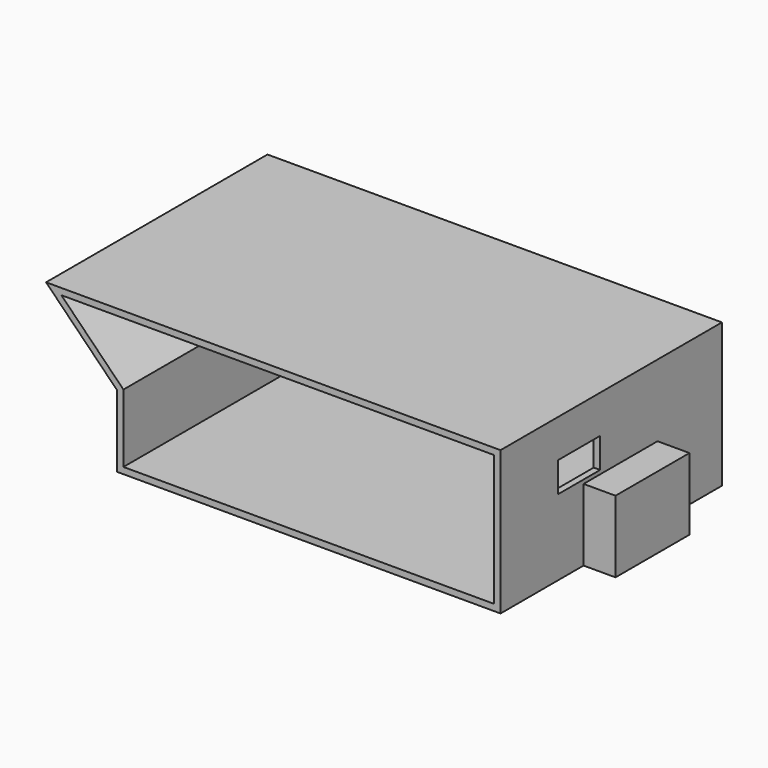
from build123d import *

# Parameters (mm, degrees)
F0_W     = 24
F0_H     = 28.575
F1_DEPTH = 54.991
F2_T     = -2.54
F3_W     = 18.5978077352
F3_H     = 17.8960040212
F4_DEPTH = 76.2
F5_W     = 36.7379160598
F5_H     = 28.575
F6_DEPTH = 12.7
F7_W     = 20.9140316583
F7_H     = 11.9311325252
F8_DEPTH = 25.4


# Not quite as in the source:
# - a feature of the source that left no trace in its solid (it failed there, or was rolled back) is left out


with BuildPart() as f1:
    # F0 (on Front) → F1 (new body, symmetric)
    with BuildSketch(Plane.XZ):
        Polygon((-76.2, -28.575), (76.2, -28.575), (76.2, 28.575), (0, 28.575), (28.2, 0), (-52.2, 0), (-76.2, 0), align=None)
        Polygon((-104.4, 28.575), (-76.2, 0), (-76.2, 28.575), align=None)
        with Locations((-64.2, 14.2875)):
            Rectangle(F0_W, F0_H)
        Polygon((28.2, 0), (0, 28.575), (-52.2, 28.575), (-52.2, 0), align=None)
    extrude(amount=F1_DEPTH, both=True)

    # F2
    f2_openings = [f1.faces().sort_by_distance(p)[0] for p in [
        (-3.78476, -54.991, 0.842286),
    ]]
    offset(amount=F2_T, openings=f2_openings, kind=Kind.INTERSECTION)

    # F3 (on Right) → F4 (join, through all)
    with BuildSketch(Plane.YZ):
        with Locations((25.7912892848, 3.5090195015)):
            Rectangle(F3_W, F3_H)
    extrude(amount=-F4_DEPTH)

    # F5 (on face) → F6 (join)
    with BuildSketch(Plane.YZ.offset(76.2)):
        with Locations((4.6260296367, -14.2875)):
            Rectangle(F5_W, F5_H)
    extrude(amount=F6_DEPTH)

    # F7 (on face) → F8 (cut)
    with BuildSketch(Plane.YZ.offset(76.2)):
        with Locations((-15.9690368455, 7.5058937073)):
            Rectangle(F7_W, F7_H)
    extrude(amount=-F8_DEPTH, mode=Mode.SUBTRACT)


solid = f1.part
